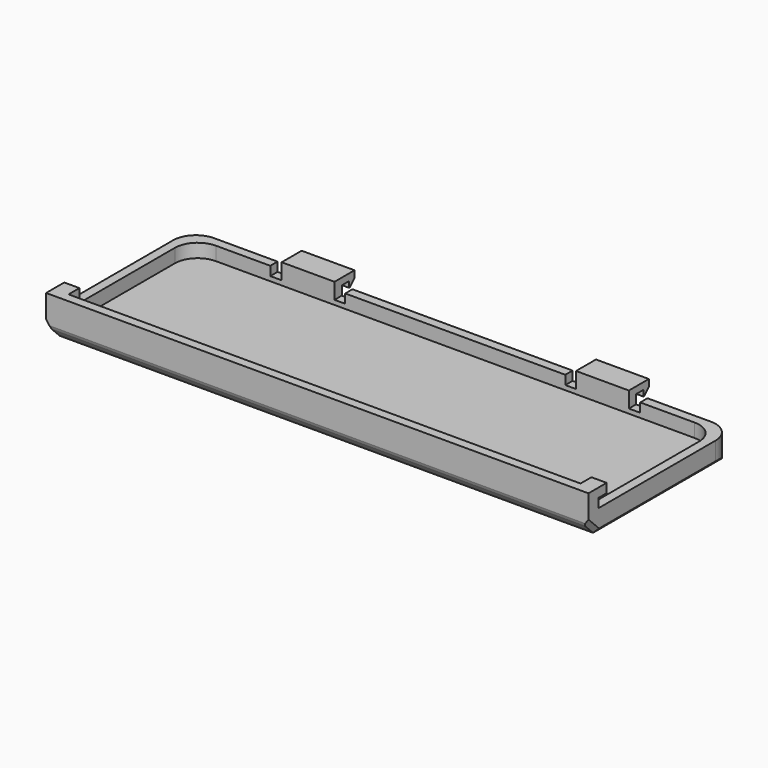
from build123d import *

# Parameters (mm, degrees)
F0_W         = 2.3
F0_H         = 2
F0_W_2       = 2
F1_DEPTH     = 119.5
F2_T         = -2
F3_DEPTH     = 3.35
F4_DEPTH     = 2.5
F5_START     = -19
F5_DEPTH     = 16.5
F6_START     = -21.5
F6_DEPTH     = 11.65
F8_W         = 11.65
F8_H         = 1
F9_DEPTH     = 0.25
F10_T1_DEPTH = 42.6433659759
F10_T3_DEPTH = 8.6788998819
F10_T5_DEPTH = 121.7571417204
F11_R        = 5


# Not quite as in the source:
# - a fillet or chamfer that OpenCascade refuses, or shapes differently, is made with other operations: its cross-section is extruded or revolved along the edge and cut away or added
# - a pattern or mirror of a feature is missing from the dataset's text; its kind, count and spacing are read off the source's solid


with BuildPart() as f1:
    # F0 (on Right) → F1 (new body)
    with BuildSketch(Plane.YZ):
        with Locations((-17.4, 6)):
            Rectangle(F0_W, F0_H)
        Polygon((-21.25, 2.5), (-20, 1.25), (-16.25, 5), (-18.55, 5), (-18.55, 7), (-16.25, 7), (-16.25, 9), (-21.25, 9), align=None)
        Polygon((-18.75, 0), (18.75, 0), (18.75, 3), (16.75, 3), (16.75, 5), (-16.25, 5), (-20, 1.25), align=None)
        with Locations((17.75, 4)):
            Rectangle(F0_W_2, F0_H)
    extrude(amount=-F1_DEPTH)

    # F2
    f2_openings = [f1.faces().sort_by_distance(p)[0] for p in [
        (-59.75, 1.25, 5),
        (-59.75, -16.25, 7),
        (-59.75, -18.75, 9),
    ]]
    offset(amount=F2_T, openings=f2_openings)

    # F0 (on Right) → F3 (join)
    with BuildSketch(Plane.YZ):
        with Locations((-17.4, 6)):
            Rectangle(F0_W, F0_H)
        Polygon((-21.25, 2.5), (-20, 1.25), (-16.25, 5), (-18.55, 5), (-18.55, 7), (-16.25, 7), (-16.25, 9), (-21.25, 9), align=None)
    f3 = extrude(amount=-F3_DEPTH)

    # F3_copies: F3 across plane
    add(f3.mirror(Plane(origin=(-59.75, 0, 0), x_dir=(0, 0, -1), z_dir=(-1, 0, 0))))

    # F0 (on Right) → F4 (cut)
    with BuildSketch(Plane.YZ):
        with Locations((-17.4, 6)):
            Rectangle(F0_W, F0_H)
    f4 = extrude(amount=-F4_DEPTH, mode=Mode.SUBTRACT)

    # F4_copies: F4 across plane
    add(f4.mirror(Plane(origin=(-59.75, 0, 0), x_dir=(0, 0, -1), z_dir=(-1, 0, 0))), mode=Mode.SUBTRACT)

    # F0 (on Right) → F5 (cut)
    with BuildSketch(Plane.YZ.offset(F5_START)):
        with Locations((17.75, 4)):
            Rectangle(F0_W_2, F0_H)
    f5 = extrude(amount=-F5_DEPTH, mode=Mode.SUBTRACT)

    # F5_copies: F5 across plane
    add(f5.mirror(Plane(origin=(-59.75, 0, 0), x_dir=(0, 0, -1), z_dir=(-1, 0, 0))), mode=Mode.SUBTRACT)

    # F0 (on Right) → F6 (join)
    with BuildSketch(Plane.YZ.offset(F6_START)):
        with Locations((17.75, 4)):
            Rectangle(F0_W_2, F0_H)
        Polygon((16.75, 5), (18.75, 5), (20.75, 5), (20.75, 3.7), (20.95, 3.7), (22.25, 5), (22.25, 6.5), (16.75, 6.5), align=None)
    f6 = extrude(amount=-F6_DEPTH)

    # F6_copies: F6 across plane
    add(f6.mirror(Plane(origin=(-59.75, 0, 0), x_dir=(0, 0, -1), z_dir=(-1, 0, 0))))

    # F8 (on face) → F9 (cut)
    with BuildSketch(Plane(origin=(0, 0, 0), x_dir=(1, 0, 0), z_dir=(0, 0, -1))):
        with Locations((-27.325, -16.25)):
            Rectangle(F8_W, F8_H)
        with Locations((-27.325, -14.25)):
            Rectangle(F8_W, F8_H)
        with Locations((-27.325, -12.25)):
            Rectangle(F8_W, F8_H)
        with Locations((-27.325, -10.25)):
            Rectangle(F8_W, F8_H)
        with Locations((-27.325, -8.25)):
            Rectangle(F8_W, F8_H)
        with Locations((-27.325, -6.25)):
            Rectangle(F8_W, F8_H)
    f9 = extrude(amount=-F9_DEPTH, mode=Mode.SUBTRACT)

    # F9_copies: F9 across plane
    add(f9.mirror(Plane(origin=(-59.75, 0, 0), x_dir=(0, 0, -1), z_dir=(-1, 0, 0))), mode=Mode.SUBTRACT)

    # F10: chamfer of 1 on 5 edges, made by hand

    # F10_s2 → F10_t1 (cut)
    with BuildSketch(Plane.XZ.offset(-21.321682988)):
        Polygon((0, 1), (-1, 0), (0, 0), align=None)
        Polygon((-119.5, 1), (-118.5, 0), (-119.5, 0), align=None)
    extrude(amount=F10_T1_DEPTH, mode=Mode.SUBTRACT)

    # F10_s4 → F10_t3 (cut)
    with BuildSketch(Plane(origin=(0, -13.6934544799, 13.6934544799), x_dir=(1, 0, 0), z_dir=(0, 0.7071067812, -0.7071067812))):
        Polygon((0, 12.2582521472), (-1, 13.2582521472), (0, 13.2582521472), align=None)
        Polygon((-119.5, 12.2582521472), (-118.5, 13.2582521472), (-119.5, 13.2582521472), align=None)
    extrude(amount=F10_T3_DEPTH, mode=Mode.SUBTRACT)

    # F10_s6 → F10_t5 (cut)
    with BuildSketch(Plane.YZ.offset(-120.6285708602)):
        Polygon((-21.25, 2.9142135624), (-20.9571067812, 2.2071067812), (-21.25, 2.5), align=None)
    extrude(amount=F10_T5_DEPTH, mode=Mode.SUBTRACT)

    # F11
    f11_edges = [f1.edges().sort_by_distance(p)[0] for p in [
        (0, 18.75, 3),
        (-119.5, 18.75, 3),
        (-2, 16.75, 3.5),
        (-117.5, 16.75, 3.5),
    ]]
    fillet(f11_edges, radius=F11_R)


solid = f1.part
